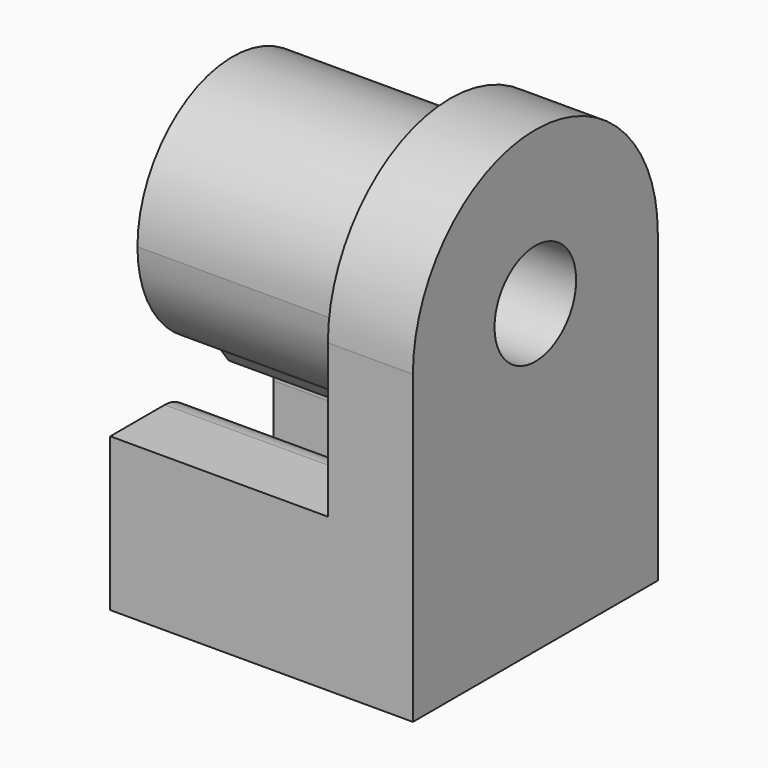
from build123d import *
from build123d import SkipClean  # not in build123d's __all__

# Parameters (mm, degrees)
F1_DEPTH = 2.5
F2_W     = 3
F2_H     = 4.5
F3_DEPTH = 6.4
F4_R     = 1
F5_R     = 0.2


with BuildPart() as f1:
    # F0 (on Right) → F1 (new body)
    with BuildSketch(Plane.YZ):
        with BuildLine():
            ThreePointArc((-4.5, 4.5), (0, 0), (4.5, 4.5))
            Line((4.5, 4.5), (1.5, 4.5))
            ThreePointArc((1.5, 4.5), (0, 3), (-1.5, 4.5))
            Line((-1.5, 4.5), (-4.5, 4.5))
        make_face()
        with BuildLine():
            Line((1.5, 4.5), (4.5, 4.5))
            ThreePointArc((4.5, 4.5), (0, 9), (-4.5, 4.5))
            Line((-4.5, 4.5), (-1.5, 4.5))
            ThreePointArc((-1.5, 4.5), (0, 6), (1.5, 4.5))
        make_face()
        with BuildLine():
            Line((-4.5, -4.5), (4.5, -4.5))
            Line((4.5, -4.5), (4.5, 4.5))
            ThreePointArc((4.5, 4.5), (0, 0), (-4.5, 4.5))
            Line((-4.5, 4.5), (-4.5, -4.5))
        make_face()
    extrude(amount=F1_DEPTH)

    # F2 (on face) → F3 (join)
    with BuildSketch(Plane(origin=(0, 0, 0), x_dir=(0, -1, 0), z_dir=(-1, 0, 0))):
        with BuildLine():
            ThreePointArc((0.8237365529, 1.0983154039), (2.7507342597, 2.3358694512), (3.5, 4.5))
            ThreePointArc((3.5, 4.5), (-2.1641305488, 7.2507342597), (-0.8237365529, 1.0983154039))
            Line((-0.8237365529, 1.0983154039), (-1.5, 2))
            Line((-1.5, 2), (0, 2))
            Line((0, 2), (1.5, 2))
            Line((1.5, 2), (0.8237365529, 1.0983154039))
        make_face()
        with BuildLine():
            ThreePointArc((1.5, 4.5), (1.0606601718, 3.4393398282), (0, 3))
            ThreePointArc((0, 3), (-1.0606601718, 5.5606601718), (1.5, 4.5))
        make_face(mode=Mode.SUBTRACT)
        with BuildLine():
            Line((-1.5, 2), (-0.8237365529, 1.0983154039))
            ThreePointArc((-0.8237365529, 1.0983154039), (-0.4147914618, 1.0246657653), (0, 1))
            Line((0, 1), (0, 2))
            Line((0, 2), (-1.5, 2))
        make_face()
        with BuildLine():
            ThreePointArc((0, 1), (-0.4147914618, 1.0246657653), (-0.8237365529, 1.0983154039))
            Line((-0.8237365529, 1.0983154039), (0, 0))
            Line((0, 0), (0, 1))
        make_face()
        with BuildLine():
            Line((0, 0), (0.8237365529, 1.0983154039))
            ThreePointArc((0.8237365529, 1.0983154039), (0.4147914618, 1.0246657653), (0, 1))
            Line((0, 1), (0, 0))
        make_face()
        with BuildLine():
            ThreePointArc((0, 1), (0.4147914618, 1.0246657653), (0.8237365529, 1.0983154039))
            Line((0.8237365529, 1.0983154039), (1.5, 2))
            Line((1.5, 2), (0, 2))
            Line((0, 2), (0, 1))
        make_face()
        with Locations((-3, -2.25)):
            Rectangle(F2_W, F2_H)
        with Locations((3, -2.25)):
            Rectangle(F2_W, F2_H)
    with SkipClean():  # cleaning this boolean's faces spoils the solid; the shape is the same uncleaned
        extrude(amount=F3_DEPTH)

    # F4
    f4_edges = [f1.edges().sort_by_distance(p)[0] for p in [
        (-3.2, 1.5, 0),
        (-3.2, -1.5, 0),
        (-3.2, 0.823737, 1.098315),
        (-3.2, -0.823737, 1.098315),
    ]]
    fillet(f4_edges, radius=F4_R)

    # F5
    f5_edges = [f1.edges().sort_by_distance(p)[0] for p in [
        (-3.2, 0, 0),
    ]]
    fillet(f5_edges, radius=F5_R)


solid = f1.part
